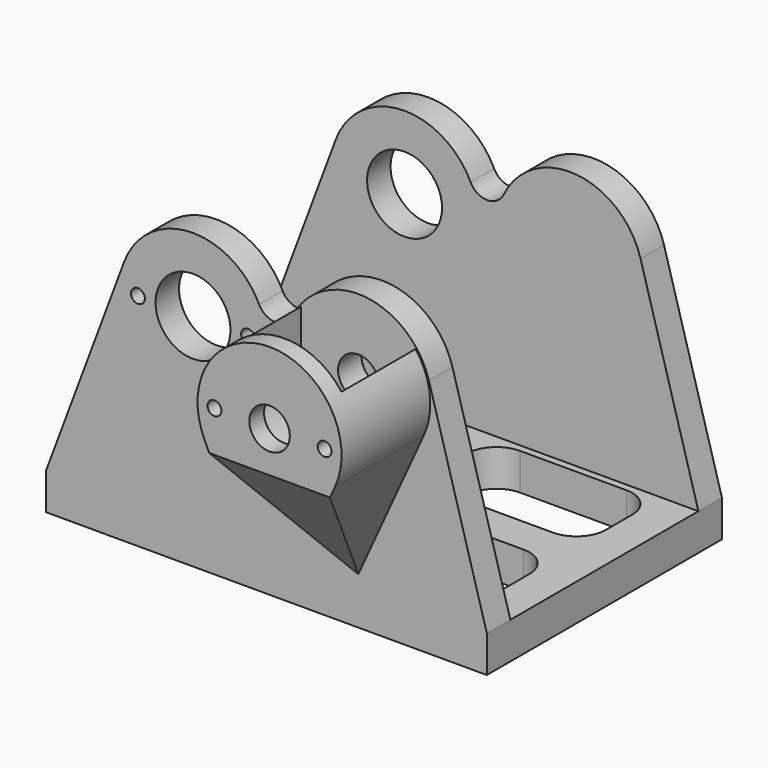
from build123d import *

# Parameters (mm, degrees)
F0_W           = 76.2
F0_H           = 50.8
F1_DEPTH       = 6.35
F2_W           = 76.2
F2_H           = 5.08
F3_DEPTH       = 101.6
F4_R           = 6.477
F5_DEPTH       = 50.801
F4_R_2         = 1.2
F4_R_3         = 3.5
F6_DEPTH       = 5.08
F8_DEPTH       = 16.002
F9_R           = 12.446
F9_R_2         = 1.2
F9_R_3         = 3.5
F10_DEPTH      = 3.175
F12_DEPTH      = 19.177
F14_DEPTH      = 38.101
F14_DEPTH_BACK = 38.101


# Not quite as in the source:
# - a feature names something its author has since deleted; it is built from what else it names


with BuildPart() as f1:
    # F0 (on Top) → F1 (new body)
    with BuildSketch(Plane.XY):
        Rectangle(F0_W, F0_H)
        with BuildLine():
            ThreePointArc((-31.75, -8.255), (-30.2621024484, -4.6628975516), (-26.67, -3.175))
            Line((-26.67, -3.175), (-8.255, -3.175))
            ThreePointArc((-8.255, -3.175), (-4.6628975516, -4.6628975516), (-3.175, -8.255))
            Line((-3.175, -8.255), (-3.175, -13.97))
            ThreePointArc((-3.175, -13.97), (-4.6628975516, -17.5621024484), (-8.255, -19.05))
            Line((-8.255, -19.05), (-26.67, -19.05))
            ThreePointArc((-26.67, -19.05), (-30.2621024484, -17.5621024484), (-31.75, -13.97))
            Line((-31.75, -13.97), (-31.75, -8.255))
        make_face(mode=Mode.SUBTRACT)
        with BuildLine():
            ThreePointArc((8.255, -19.05), (4.6628975516, -17.5621024484), (3.175, -13.97))
            Line((3.175, -13.97), (3.175, -8.255))
            ThreePointArc((3.175, -8.255), (4.6628975516, -4.6628975516), (8.255, -3.175))
            Line((8.255, -3.175), (26.67, -3.175))
            ThreePointArc((26.67, -3.175), (30.2621024484, -4.6628975516), (31.75, -8.255))
            Line((31.75, -8.255), (31.75, -13.97))
            ThreePointArc((31.75, -13.97), (30.2621024484, -17.5621024484), (26.67, -19.05))
            Line((26.67, -19.05), (8.255, -19.05))
        make_face(mode=Mode.SUBTRACT)
        with BuildLine():
            ThreePointArc((-31.75, 13.97), (-30.2621024484, 17.5621024484), (-26.67, 19.05))
            Line((-26.67, 19.05), (-8.255, 19.05))
            ThreePointArc((-8.255, 19.05), (-4.6628975516, 17.5621024484), (-3.175, 13.97))
            Line((-3.175, 13.97), (-3.175, 8.255))
            ThreePointArc((-3.175, 8.255), (-4.6628975516, 4.6628975516), (-8.255, 3.175))
            Line((-8.255, 3.175), (-26.67, 3.175))
            ThreePointArc((-26.67, 3.175), (-30.2621024484, 4.6628975516), (-31.75, 8.255))
            Line((-31.75, 8.255), (-31.75, 13.97))
        make_face(mode=Mode.SUBTRACT)
        with BuildLine():
            Line((31.75, 13.97), (31.75, 8.255))
            ThreePointArc((31.75, 8.255), (30.2621024484, 4.6628975516), (26.67, 3.175))
            Line((26.67, 3.175), (8.255, 3.175))
            ThreePointArc((8.255, 3.175), (4.6628975516, 4.6628975516), (3.175, 8.255))
            Line((3.175, 8.255), (3.175, 13.97))
            ThreePointArc((3.175, 13.97), (4.6628975516, 17.5621024484), (8.255, 19.05))
            Line((8.255, 19.05), (26.67, 19.05))
            ThreePointArc((26.67, 19.05), (30.2621024484, 17.5621024484), (31.75, 13.97))
        make_face(mode=Mode.SUBTRACT)
    extrude(amount=F1_DEPTH)

    # F2 (on face) → F3 (join)
    with BuildSketch(Plane.XY.offset(6.35)):
        with Locations((0, 22.86)):
            Rectangle(F2_W, F2_H)
        with Locations((0, -22.86)):
            Rectangle(F2_W, F2_H)
    extrude(amount=F3_DEPTH)

    # F4 (on face) → F5 (cut, through all)
    with BuildSketch(Plane.XZ.offset(25.4)):
        with BuildLine():
            Line((28.0908644484, 41.5545914238), (38.1, 6.35))
            Line((38.1, 6.35), (38.1, 107.95))
            Line((38.1, 107.95), (-38.1, 107.95))
            Line((-38.1, 107.95), (-38.1, 6.35))
            Line((-38.1, 6.35), (-24.5981673582, 42.522585505))
            ThreePointArc((-24.5981673582, 42.522585505), (-13.2952924023, 50.7674986335), (-1.27, 43.6172596583))
            ThreePointArc((-1.27, 43.6172596583), (1.5875, 41.8262100729), (4.445, 43.6172596583))
            ThreePointArc((4.445, 43.6172596583), (16.9786511198, 50.7334125607), (28.0908644484, 41.5545914238))
        make_face()
        with Locations((-12.7, 38.081458)):
            Circle(F4_R)
    extrude(amount=-F5_DEPTH, mode=Mode.SUBTRACT)

    # F4 (on face) → F6 (cut, through all)
    with BuildSketch(Plane.XZ.offset(25.4)):
        with Locations((-3.175, 38.081458)):
            Circle(F4_R_2)
        with Locations((-22.225, 38.081458)):
            Circle(F4_R_2)
        with Locations((15.875, 38.081458)):
            Circle(F4_R_3)
    extrude(amount=-F6_DEPTH, mode=Mode.SUBTRACT)

    # F7 (on face) → F8 (join)
    with BuildSketch(Plane.XZ.offset(25.4)):
        with BuildLine():
            ThreePointArc((25.781, 38.081458), (15.875, 28.175458), (5.969, 38.081458))
            Line((5.969, 38.081458), (5.969, 45.6163156629))
            ThreePointArc((5.969, 45.6163156629), (15.875, 25.635458), (25.781, 45.6163156629))
            Line((25.781, 45.6163156629), (25.781, 38.081458))
        make_face()
    extrude(amount=F8_DEPTH)

    # F9 (on face) → F10 (join)
    with BuildSketch(Plane.XZ.offset(41.402)):
        with Locations((15.875, 38.081458)):
            Circle(F9_R)
        with Locations((6.35, 38.081458)):
            Circle(F9_R_2, mode=Mode.SUBTRACT)
        with Locations((15.875, 38.081458)):
            Circle(F9_R_3, mode=Mode.SUBTRACT)
        with Locations((25.4, 38.081458)):
            Circle(F9_R_2, mode=Mode.SUBTRACT)
    extrude(amount=F10_DEPTH)

    # F11 (on face) → F12 (join, through all)
    with BuildSketch(Plane.XZ.offset(25.4)):
        with BuildLine():
            Line((4.5542674961, 32.9100044737), (15.875, 8.128))
            Line((15.875, 8.128), (27.1957325039, 32.9100044737))
            ThreePointArc((27.1957325039, 32.9100044737), (15.875, 25.635458), (4.5542674961, 32.9100044737))
        make_face()
    extrude(amount=F12_DEPTH)

    # F13 (on Right) → F14 (cut, two sides)
    with BuildSketch(Plane.YZ) as f14_sk:
        Polygon((-25.4, 8.128), (-44.577, 30.9822586452), (-44.577, 8.128), align=None)
    extrude(amount=-F14_DEPTH, mode=Mode.SUBTRACT)
    extrude(f14_sk.sketch, amount=F14_DEPTH_BACK, mode=Mode.SUBTRACT)


solid = f1.part
